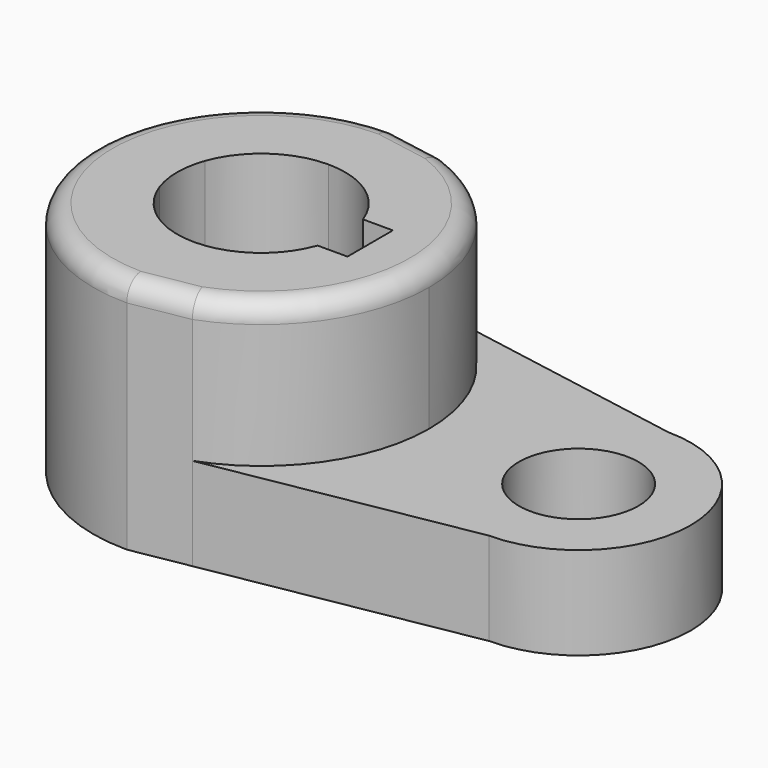
from build123d import *

# Parameters (mm, degrees)
F0_R        = 10.16
F1_DEPTH    = 15.7734
F2_DEPTH    = 40.2336
F3_T1_DEPTH = 37.9988318329
F3_T3_DEPTH = 37.9988318329
F3_T6_ANGLE = 213.1574660215
F3_T8_ANGLE = 173.1044855741


# Not quite as in the source:
# - a fillet or chamfer that OpenCascade refuses, or shapes differently, is made with other operations: its cross-section is extruded or revolved along the edge and cut away or added


with BuildPart() as f1:
    # F0 (on Top) → F1 (new body)
    with BuildSketch(Plane.XY):
        with BuildLine():
            Line((53.975, 19.05), (9.780704698, 26.8489932886))
            ThreePointArc((9.780704698, 26.8489932886), (23.4095521288, 16.3866864902), (28.575, 0))
            ThreePointArc((28.575, 0), (23.4095521288, -16.3866864902), (9.780704698, -26.8489932886))
            Line((9.780704698, -26.8489932886), (53.975, -19.05))
            ThreePointArc((53.975, -19.05), (73.025, 0), (53.975, 19.05))
        make_face()
        with Locations((53.975, 0)):
            Circle(F0_R, mode=Mode.SUBTRACT)
    extrude(amount=F1_DEPTH)

    # F0 (on Top) → F2 (join)
    with BuildSketch(Plane.XY):
        with BuildLine():
            Line((9.780704698, 26.8489932886), (0, 28.575))
            ThreePointArc((0, 28.575), (-28.575, 0), (0, -28.575))
            Line((0, -28.575), (9.780704698, -26.8489932886))
            ThreePointArc((9.780704698, -26.8489932886), (23.4095521288, -16.3866864902), (28.575, 0))
            ThreePointArc((28.575, 0), (23.4095521288, 16.3866864902), (9.780704698, 26.8489932886))
        make_face()
        with BuildLine():
            ThreePointArc((-13.4477648793, 4.826), (-8.2213496839, 11.6851215494), (0, 14.2875))
            ThreePointArc((0, 14.2875), (8.2213496839, 11.6851215494), (13.4477648793, 4.826))
            Line((13.4477648793, 4.826), (18.5293, 4.826))
            Line((18.5293, 4.826), (18.5293, -4.826))
            Line((18.5293, -4.826), (13.4477648793, -4.826))
            ThreePointArc((13.4477648793, -4.826), (0, -14.2875), (-13.4477648793, -4.826))
            Line((-13.4477648793, -4.826), (-18.5293, -4.826))
            Line((-18.5293, -4.826), (-18.5293, 4.826))
            Line((-18.5293, 4.826), (-13.4477648793, 4.826))
        make_face(mode=Mode.SUBTRACT)
        with BuildLine():
            ThreePointArc((-13.4477648793, -4.826), (-14.2875, 0), (-13.4477648793, 4.826))
            Line((-13.4477648793, 4.826), (-18.5293, 4.826))
            Line((-18.5293, 4.826), (-18.5293, -4.826))
            Line((-18.5293, -4.826), (-13.4477648793, -4.826))
        make_face()
    extrude(amount=F2_DEPTH)

    # F3: fillet of radius 3.302 on 4 edges, made by hand

    # F3_s2 → F3_t1 (cut)
    with BuildSketch(Plane(origin=(18.7103124217, -3.3018198391, 0), x_dir=(0, 0, 1), z_dir=(-0.9847835588, 0.1737853339, 0))):
        with BuildLine():
            ThreePointArc((36.9316, 28.1401901932), (39.2664665915, 27.1730567847), (40.2336, 24.8381901932))
            Line((40.2336, 24.8381901932), (40.2336, 28.1401901932))
            Line((40.2336, 28.1401901932), (36.9316, 28.1401901932))
        make_face()
    extrude(amount=F3_T1_DEPTH, mode=Mode.SUBTRACT)

    # F3_s4 → F3_t3 (cut)
    with BuildSketch(Plane(origin=(-18.7103124217, -3.3018198391, 0), x_dir=(0, 0, 1), z_dir=(0.9847835588, 0.1737853339, 0))):
        with BuildLine():
            ThreePointArc((36.9316, 28.1401901932), (39.2664665915, 27.1730567847), (40.2336, 24.8381901932))
            Line((40.2336, 24.8381901932), (40.2336, 28.1401901932))
            Line((40.2336, 28.1401901932), (36.9316, 28.1401901932))
        make_face()
    extrude(amount=F3_T3_DEPTH, mode=Mode.SUBTRACT)

    # F3_s5 → F3_t6 (revolve, cut)
    with BuildSketch(Plane(origin=(0, 0, 0), x_dir=(0, 0, 1), z_dir=(0.95842855, -0.2853326385, 0))):
        with BuildLine():
            ThreePointArc((40.2336, -25.273), (39.2664665915, -27.6078665915), (36.9316, -28.575))
            Line((36.9316, -28.575), (40.2336, -28.575))
            Line((40.2336, -28.575), (40.2336, -25.273))
        make_face()
    revolve(axis=Axis((0, 0, 40.2336), (0, 0, 1)), revolution_arc=F3_T6_ANGLE, mode=Mode.SUBTRACT)

    # F3_s7 → F3_t8 (revolve, cut)
    with BuildSketch(Plane(origin=(0, 0, 0), x_dir=(0, 0, 1), z_dir=(-0.9981900481, -0.0601384063, 0))):
        with BuildLine():
            ThreePointArc((36.9316, -28.575), (39.2664665915, -27.6078665915), (40.2336, -25.273))
            Line((40.2336, -25.273), (40.2336, -28.575))
            Line((40.2336, -28.575), (36.9316, -28.575))
        make_face()
    revolve(axis=Axis((0, 0, 40.2336), (0, 0, 1)), revolution_arc=F3_T8_ANGLE, mode=Mode.SUBTRACT)


solid = f1.part
